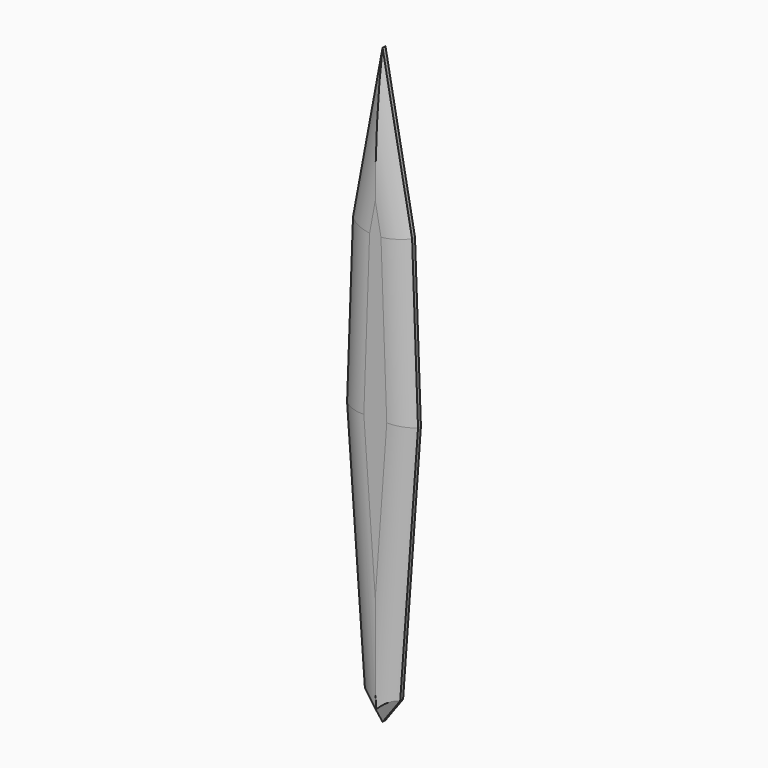
from build123d import *

# Parameters (mm, degrees)
F1_DEPTH     = 7.62
F2_DEPTH     = 7.62
F3_SIZE2     = 6.35
F3_SIZE      = 6.35
F4_T1_DEPTH  = 327.4383964473
F4_T3_DEPTH  = 323.6073894147
F4_T5_DEPTH  = 201.3367308849
F4_T7_DEPTH  = 201.3367308849
F4_T9_DEPTH  = 327.4383964473
F4_T11_DEPTH = 323.6073894147
F4_T13_DEPTH = 327.4383964473
F4_T15_DEPTH = 327.4383964473
F4_T20_DEPTH = 62.7434560732
F4_S21_R     = 25.4
F4_T22_DEPTH = 41
F4_T26_DEPTH = 62.7434560732
F4_S27_R     = 25.4
F4_T28_DEPTH = 41
F4_T32_DEPTH = 62.7434560732
F4_S33_R     = 25.4
F4_T34_DEPTH = 41
F4_T38_DEPTH = 62.7434560732
F4_S39_R     = 25.4
F4_T40_DEPTH = 41


# Not quite as in the source:
# - a fillet or chamfer that OpenCascade refuses, or shapes differently, is made with other operations: its cross-section is extruded or revolved along the edge and cut away or added


with BuildPart() as f1:
    # F0 (on Front) → F1 (new body)
    with BuildSketch(Plane.XZ):
        Polygon((20.717933774, 293.1892871857), (0, 404.365837574), (-20.717933774, 293.1892871857), (-24.8540937901, 177.8507977724), (-17.5723880529, 77.2872418165), (-12.3717649418, 5.4643513949), (0, -11.5514695644), (12.3717649418, 5.4643513949), (17.5723880529, 77.2872418165), (24.8540937901, 177.8507977724), align=None)
    extrude(amount=F1_DEPTH)

    # F2 (add): a face of the model
    f2_faces = [f1.faces().sort_by_distance(p)[0] for p in [
        (0, 0, 186.0406661008),
    ]]
    extrude(f2_faces, amount=F2_DEPTH)

    # F3
    f3_edges = [f1.edges().sort_by_distance(p)[0] for p in [
        (18.612929, -7.62, 91.657575),
        (22.786014, -7.62, 235.520042),
        (10.358967, -7.62, 348.777562),
        (-10.358967, -7.62, 348.777562),
        (-22.786014, -7.62, 235.520042),
        (-18.612929, -7.62, 91.657575),
        (-6.185882, -7.62, -3.043559),
        (6.185882, -7.62, -3.043559),
        (22.786014, 7.62, 235.520042),
        (10.358967, 7.62, 348.777562),
        (-10.358967, 7.62, 348.777562),
        (-22.786014, 7.62, 235.520042),
        (-18.612929, 7.62, 91.657575),
        (-6.185882, 7.62, -3.043559),
        (6.185882, 7.62, -3.043559),
        (18.612929, 7.62, 91.657575),
    ]]
    chamfer(f3_edges, length=F3_SIZE, length2=F3_SIZE2)

    # F4: fillet of radius 25.4 on 16 edges, made by hand

    # F4_s2 → F4_t1 (cut)
    with BuildSketch(Plane(origin=(22.3498393806, 0, 308.6611028095), x_dir=(0, 1, 0), z_dir=(-0.072219913, 0, -0.9973887327))):
        with BuildLine():
            ThreePointArc((-1.27, 11.9448239749), (-5.979524406, 4.1245592707), (-7.62, -4.8556968504))
            Line((-7.62, -4.8556968504), (-7.62, 5.5948239749))
            Line((-7.62, 5.5948239749), (-1.27, 11.9448239749))
        make_face()
    extrude(amount=F4_T1_DEPTH, mode=Mode.SUBTRACT)

    # F4_s4 → F4_t3 (cut)
    with BuildSketch(Plane(origin=(-1.668545053, 0, 46.5280514247), x_dir=(0, 1, 0), z_dir=(-0.0358380192, 0, 0.9993576119))):
        with BuildLine():
            ThreePointArc((-1.27, -31.2119481169), (-5.979524406, -23.3916834127), (-7.62, -14.4114272916))
            Line((-7.62, -14.4114272916), (-7.62, -24.8619481169))
            Line((-7.62, -24.8619481169), (-1.27, -31.2119481169))
        make_face()
        with BuildLine():
            ThreePointArc((1.27, -31.2119481169), (5.979524406, -23.3916834127), (7.62, -14.4114272916))
            Line((7.62, -14.4114272916), (7.62, -24.8619481169))
            Line((7.62, -24.8619481169), (1.27, -31.2119481169))
        make_face()
    extrude(amount=F4_T3_DEPTH, mode=Mode.SUBTRACT)

    # F4_s6 → F4_t5 (cut)
    with BuildSketch(Plane(origin=(-37.8349349921, 0, 203.0297809848), x_dir=(0, 1, 0), z_dir=(-0.1831978482, 0, 0.9830760644))):
        with BuildLine():
            ThreePointArc((-7.62, -57.2784304891), (-5.979524406, -66.2586866102), (-1.27, -74.0789513144))
            Line((-1.27, -74.0789513144), (-7.62, -67.7289513144))
            Line((-7.62, -67.7289513144), (-7.62, -57.2784304891))
        make_face()
        with BuildLine():
            ThreePointArc((7.62, -57.2784304891), (5.979524406, -66.2586866102), (1.27, -74.0789513144))
            Line((1.27, -74.0789513144), (7.62, -67.7289513144))
            Line((7.62, -67.7289513144), (7.62, -57.2784304891))
        make_face()
    extrude(amount=F4_T5_DEPTH, mode=Mode.SUBTRACT)

    # F4_s8 → F4_t7 (cut)
    with BuildSketch(Plane(origin=(74.7193908465, 0, 400.9591020056), x_dir=(0, 1, 0), z_dir=(-0.1831978482, 0, -0.9830760644))):
        with BuildLine():
            ThreePointArc((-7.62, -57.2784304891), (-5.979524406, -66.2586866102), (-1.27, -74.0789513144))
            Line((-1.27, -74.0789513144), (-7.62, -67.7289513144))
            Line((-7.62, -67.7289513144), (-7.62, -57.2784304891))
        make_face()
        with BuildLine():
            ThreePointArc((7.62, -57.2784304891), (5.979524406, -66.2586866102), (1.27, -74.0789513144))
            Line((1.27, -74.0789513144), (7.62, -67.7289513144))
            Line((7.62, -67.7289513144), (7.62, -57.2784304891))
        make_face()
    extrude(amount=F4_T7_DEPTH, mode=Mode.SUBTRACT)

    # F4_s10 → F4_t9 (cut)
    with BuildSketch(Plane(origin=(1.2977331079, 0, -17.9222644696), x_dir=(0, 1, 0), z_dir=(-0.072219913, 0, 0.9973887327))):
        with BuildLine():
            ThreePointArc((-7.62, -4.8556968504), (-5.979524406, 4.1245592707), (-1.27, 11.9448239749))
            Line((-1.27, 11.9448239749), (-7.62, 5.5948239749))
            Line((-7.62, 5.5948239749), (-7.62, -4.8556968504))
        make_face()
    extrude(amount=F4_T9_DEPTH, mode=Mode.SUBTRACT)

    # F4_s12 → F4_t11 (cut)
    with BuildSketch(Plane(origin=(13.265992882, 0, 369.9275592901), x_dir=(0, 1, 0), z_dir=(-0.0358380192, 0, -0.9993576119))):
        with BuildLine():
            ThreePointArc((-7.62, -14.4114272916), (-5.979524406, -23.3916834127), (-1.27, -31.2119481169))
            Line((-1.27, -31.2119481169), (-7.62, -24.8619481169))
            Line((-7.62, -24.8619481169), (-7.62, -14.4114272916))
        make_face()
        with BuildLine():
            ThreePointArc((7.62, -14.4114272916), (5.979524406, -23.3916834127), (1.27, -31.2119481169))
            Line((1.27, -31.2119481169), (7.62, -24.8619481169))
            Line((7.62, -24.8619481169), (7.62, -14.4114272916))
        make_face()
    extrude(amount=F4_T11_DEPTH, mode=Mode.SUBTRACT)

    # F4_s14 → F4_t13 (cut)
    with BuildSketch(Plane(origin=(-1.2977331079, 0, -17.9222644696), x_dir=(0, 1, 0), z_dir=(0.072219913, 0, 0.9973887327))):
        with BuildLine():
            ThreePointArc((1.27, -11.9448239749), (5.979524406, -4.1245592707), (7.62, 4.8556968504))
            Line((7.62, 4.8556968504), (7.62, -5.5948239749))
            Line((7.62, -5.5948239749), (1.27, -11.9448239749))
        make_face()
    extrude(amount=F4_T13_DEPTH, mode=Mode.SUBTRACT)

    # F4_s16 → F4_t15 (cut)
    with BuildSketch(Plane(origin=(-22.3498393806, 0, 308.6611028095), x_dir=(0, 1, 0), z_dir=(0.072219913, 0, -0.9973887327))):
        with BuildLine():
            ThreePointArc((7.62, 4.8556968504), (5.979524406, -4.1245592707), (1.27, -11.9448239749))
            Line((1.27, -11.9448239749), (7.62, -5.5948239749))
            Line((7.62, -5.5948239749), (7.62, 4.8556968504))
        make_face()
    extrude(amount=F4_T15_DEPTH, mode=Mode.SUBTRACT)


with BuildPart() as f4_tool18:
    # F4_s19 → F4_t20 (new body)
    with BuildSketch(Plane(origin=(-15.7223396598, 0, -21.6241189491), x_dir=(0, 1, 0), z_dir=(0.5880666869, 0, 0.8088124454))):
        with BuildLine():
            ThreePointArc((-7.62, 10.0074863899), (-5.979524406, 1.0272302688), (-1.27, -6.7930344354))
            Line((-1.27, -6.7930344354), (-7.62, -0.4430344354))
            Line((-7.62, -0.4430344354), (-7.62, 10.0074863899))
        make_face()
    extrude(amount=F4_T20_DEPTH)

    # F4_s21 → F4_t22 (cut, symmetric)
    with BuildSketch(Plane(origin=(0.3466555822, 0, 4.7874659171), x_dir=(0, 1, 0), z_dir=(0.072219913, 0, 0.9973887327))):
        with Locations((17.78, 4.8556968504)):
            Circle(F4_S21_R)
    extrude(amount=F4_T22_DEPTH, both=True, mode=Mode.SUBTRACT)


with BuildPart() as f1_1:
    add(f1.part)

    # F4_t17: cut F4_tool18
    add(f4_tool18.part, mode=Mode.SUBTRACT)


with BuildPart() as f4_tool24:
    # F4_s25 → F4_t26 (new body)
    with BuildSketch(Plane(origin=(-21.1749966767, 0, 29.1235691883), x_dir=(0, 1, 0), z_dir=(0.5880666869, 0, -0.8088124454))):
        with BuildLine():
            ThreePointArc((-7.62, 10.0074863899), (-5.979524406, 1.0272302688), (-1.27, -6.7930344354))
            Line((-1.27, -6.7930344354), (-7.62, -0.4430344354))
            Line((-7.62, -0.4430344354), (-7.62, 10.0074863899))
        make_face()
    extrude(amount=F4_T26_DEPTH)

    # F4_s27 → F4_t28 (cut, symmetric)
    with BuildSketch(Plane(origin=(-0.3466555822, 0, 4.7874659171), x_dir=(0, 1, 0), z_dir=(0.072219913, 0, -0.9973887327))):
        with Locations((17.78, 4.8556968504)):
            Circle(F4_S27_R)
    extrude(amount=F4_T28_DEPTH, both=True, mode=Mode.SUBTRACT)


with BuildPart() as f1_2:
    add(f1_1.part)

    # F4_t23: cut F4_tool24
    add(f4_tool24.part, mode=Mode.SUBTRACT)


with BuildPart() as f4_tool30:
    # F4_s31 → F4_t32 (new body)
    with BuildSketch(Plane(origin=(-15.7223396598, 0, -21.6241189491), x_dir=(0, 1, 0), z_dir=(0.5880666869, 0, 0.8088124454))):
        with BuildLine():
            ThreePointArc((1.27, -6.7930344354), (5.979524406, 1.0272302688), (7.62, 10.0074863899))
            Line((7.62, 10.0074863899), (7.62, -0.4430344354))
            Line((7.62, -0.4430344354), (1.27, -6.7930344354))
        make_face()
    extrude(amount=F4_T32_DEPTH)

    # F4_s33 → F4_t34 (cut, symmetric)
    with BuildSketch(Plane(origin=(0.3466555822, 0, 4.7874659171), x_dir=(0, 1, 0), z_dir=(-0.072219913, 0, -0.9973887327))):
        with Locations((-17.78, -4.8556968504)):
            Circle(F4_S33_R)
    extrude(amount=F4_T34_DEPTH, both=True, mode=Mode.SUBTRACT)


with BuildPart() as f1_3:
    add(f1_2.part)

    # F4_t29: cut F4_tool30
    add(f4_tool30.part, mode=Mode.SUBTRACT)


with BuildPart() as f4_tool36:
    # F4_s37 → F4_t38 (new body)
    with BuildSketch(Plane(origin=(-21.1749966767, 0, 29.1235691883), x_dir=(0, 1, 0), z_dir=(0.5880666869, 0, -0.8088124454))):
        with BuildLine():
            ThreePointArc((7.62, 10.0074863899), (5.979524406, 1.0272302688), (1.27, -6.7930344354))
            Line((1.27, -6.7930344354), (7.62, -0.4430344354))
            Line((7.62, -0.4430344354), (7.62, 10.0074863899))
        make_face()
    extrude(amount=F4_T38_DEPTH)

    # F4_s39 → F4_t40 (cut, symmetric)
    with BuildSketch(Plane(origin=(-0.3466555822, 0, 4.7874659171), x_dir=(0, 1, 0), z_dir=(-0.072219913, 0, 0.9973887327))):
        with Locations((-17.78, -4.8556968504)):
            Circle(F4_S39_R)
    extrude(amount=F4_T40_DEPTH, both=True, mode=Mode.SUBTRACT)


with BuildPart() as f1_4:
    add(f1_3.part)

    # F4_t35: cut F4_tool36
    add(f4_tool36.part, mode=Mode.SUBTRACT)


solid = f1_4.part
